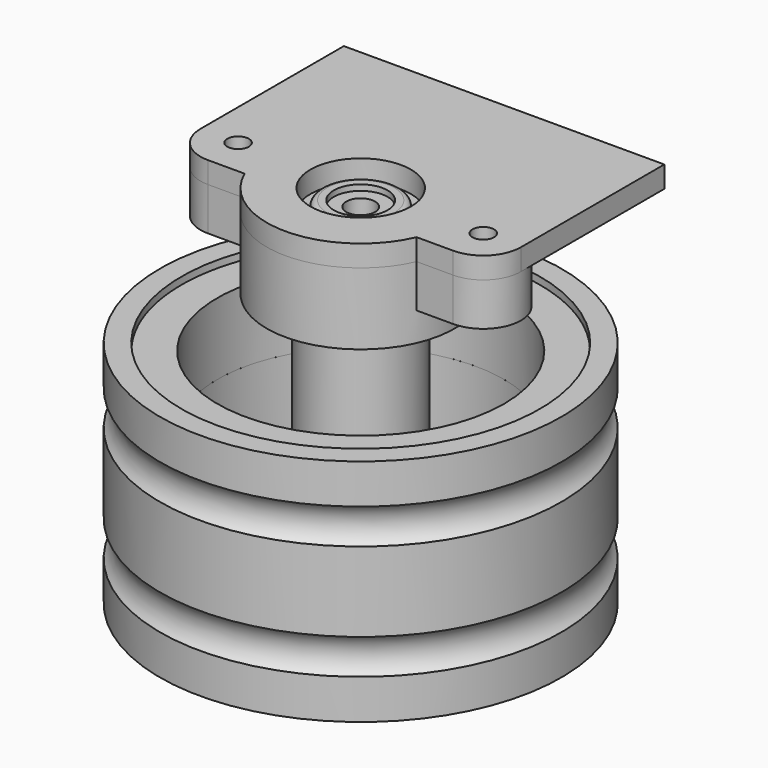
from build123d import *

# Parameters (mm, degrees)
F4_R           = 7.5
F4_R_2         = 3.75
F4_R_3         = 2.25
F5_DEPTH       = 10
F6_DEPTH       = 7.5
F9_W           = 2.45
F9_H           = 5
F11_R          = 0.2
F11_2_R        = 0.2
F12_R          = 0.6
F12_2_R        = 0.6
F13_R          = 0.8
F18_R          = 3.75
F18_R_2        = 2
F19_DEPTH      = 2
F20_DEPTH      = 6
F22_COUNT      = 2
F2_W           = 2
F2_H           = 5
F27_R          = 1.5
F28_REACH      = 54.2436406871
F31_END_RADIUS = 20
F30_R          = 3.5
F30_R_2        = 1.5
F31_REACH      = 16.9004949366
F27_R_2        = 2
F35_R          = 2
F36_DEPTH      = 47.1000001314
F38_DEPTH      = 4
F41_DEPTH      = 1
F42_R          = 2
F42_R_2        = 1.5
F43_DEPTH      = 3
F46_R          = 1


# Not quite as in the source:
# - a feature names something its author has since deleted; it is built from what else it names


with BuildPart() as f5:
    # F4 (on Top) → F5 (new body)
    with BuildSketch(Plane.XY):
        Circle(F4_R)
        Circle(F4_R_2, mode=Mode.SUBTRACT)
        Circle(F4_R_2)
        Circle(F4_R_3, mode=Mode.SUBTRACT)
    extrude(amount=F5_DEPTH)

    # F4 (on Top) → F6 (cut)
    with BuildSketch(Plane.XY):
        Circle(F4_R_2)
        Circle(F4_R_3, mode=Mode.SUBTRACT)
    extrude(amount=F6_DEPTH, mode=Mode.SUBTRACT)

    # F7 (on Front) → F8 (revolve)
    with BuildSketch(Plane.XZ):
        Polygon((-4.875, 12), (-6.0297005384, 10), (-3.7202994616, 10), align=None)
    revolve(axis=Axis((0, 0, 0), (0, 0, -1)))

    # F11
    f11_edges = [f5.edges().sort_by_distance(p)[0] for p in [
        (4.875, 0, 12),
    ]]
    fillet(f11_edges, radius=F11_R)

    # F12
    f12_edges = [f5.edges().sort_by_distance(p)[0] for p in [
        (-2.25, 0, 7.5),
        (-3.75, 0, 7.5),
    ]]
    fillet(f12_edges, radius=F12_R)



with BuildPart() as f10:
    # F9 (on Front) → F10 (revolve)
    with BuildSketch(Plane.XZ):
        Polygon((1.5, 20), (1.5, 10), (3.6048294078, 10), (4.875, 12.2), (6.1451705922, 10), (7.5, 10), (7.5, 35.7358983849), (5.5, 39.2), (5.5, 40), (3.95, 40), (1.5, 40), (1.5, 37), (0, 37), (0, 20), align=None)
        with Locations((2.725, 42.5)):
            Rectangle(F9_W, F9_H)
    revolve(axis=Axis((0, 0, 27.5), (0, 0, 1)))

    # F11#2
    f11_2_edges = [f10.edges().sort_by_distance(p)[0] for p in [
        (-4.875, 0, 12.2),
    ]]
    fillet(f11_2_edges, radius=F11_2_R)

    # F12#2
    f12_2_edges = [f10.edges().sort_by_distance(p)[0] for p in [
        (-1.5, 0, 20),
    ]]
    fillet(f12_2_edges, radius=F12_2_R)


with BuildPart() as f10b:
    # F9 (on Front) → F10, piece 2 (revolve)
    with BuildSketch(Plane.XZ):
        Polygon((2, 45.2), (3.95, 45.2), (3.95, 47), (5.5, 47), (5.5, 48.5), (3.75, 48.5), (3.75, 47.7), (2, 47.7), align=None)
    revolve(axis=Axis((0, 0, 27.5), (0, 0, 1)))

    # F13
    f13_edges = [f10b.edges().sort_by_distance(p)[0] for p in [
        (-5.5, 0, 48.5),
    ]]
    fillet(f13_edges, radius=F13_R)


with BuildPart() as f15:
    # F14 (on Front) → F15 (revolve)
    with BuildSketch(Plane.XZ):
        Polygon((-5.5, 40), (-5.5, 47), (-11, 47), (-11, 43.5), (-11, 40), align=None)
        Polygon((-4, 47), (-5.5, 47), (-5.5, 40), (-4, 40), (-4, 43.5), align=None)
    revolve(axis=Axis((0, 0, 43.5), (0, 0, 1)))


with BuildPart() as f17:
    # F16 (on Front) → F17 (revolve)
    with BuildSketch(Plane.XZ):
        Polygon((-7, 38.5), (-7, 40), (-11.1, 40), (-11.1, 47), (-13.1, 47), (-13.1, 44), (-13.1, 37), (-7.8660254038, 37), align=None)
    revolve(axis=Axis((0, 0, 42.5), (0, 0, -1)))

    # F18 (on face) → F19 (join)
    with BuildSketch(Plane.XY.offset(47)):
        with BuildLine():
            ThreePointArc((-12.7619152047, 2.956944421), (-14.6465797557, 4.6414684212), (-17.1, 5.25))
            ThreePointArc((-17.1, 5.25), (-22.35, 0), (-17.1, -5.25))
            ThreePointArc((-17.1, -5.25), (-14.6465797557, -4.6414684212), (-12.7619152047, -2.956944421))
            ThreePointArc((-12.7619152047, -2.956944421), (-13.1, 0), (-12.7619152047, 2.956944421))
        make_face()
        with Locations((-17.1, 0)):
            Circle(F18_R, mode=Mode.SUBTRACT)
        with Locations((-17.1, 0)):
            Circle(F18_R)
        with Locations((-17.1, 0)):
            Circle(F18_R_2, mode=Mode.SUBTRACT)
        with BuildLine():
            ThreePointArc((-12.7619152047, -2.956944421), (-14.6465797557, -4.6414684212), (-17.1, -5.25))
            Line((-17.1, -5.25), (-12.0019790035, -5.25))
            ThreePointArc((-12.0019790035, -5.25), (-12.4349161662, -4.1210265638), (-12.7619152047, -2.956944421))
        make_face()
        with BuildLine():
            Line((-12.0019790035, 5.25), (-17.1, 5.25))
            ThreePointArc((-17.1, 5.25), (-14.6465797557, 4.6414684212), (-12.7619152047, 2.956944421))
            ThreePointArc((-12.7619152047, 2.956944421), (-12.4349161662, 4.1210265638), (-12.0019790035, 5.25))
        make_face()
    extrude(amount=-F19_DEPTH)

    # F18 (on face) → F20 (join)
    with BuildSketch(Plane.XY.offset(47)):
        with BuildLine():
            ThreePointArc((-12.7619152047, 2.956944421), (-14.6465797557, 4.6414684212), (-17.1, 5.25))
            ThreePointArc((-17.1, 5.25), (-22.35, 0), (-17.1, -5.25))
            ThreePointArc((-17.1, -5.25), (-14.6465797557, -4.6414684212), (-12.7619152047, -2.956944421))
            ThreePointArc((-12.7619152047, -2.956944421), (-13.1, 0), (-12.7619152047, 2.956944421))
        make_face()
        with Locations((-17.1, 0)):
            Circle(F18_R, mode=Mode.SUBTRACT)
        with BuildLine():
            Line((-12.0019790035, 5.25), (-17.1, 5.25))
            ThreePointArc((-17.1, 5.25), (-14.6465797557, 4.6414684212), (-12.7619152047, 2.956944421))
            ThreePointArc((-12.7619152047, 2.956944421), (-12.4349161662, 4.1210265638), (-12.0019790035, 5.25))
        make_face()
        with BuildLine():
            ThreePointArc((-12.7619152047, -2.956944421), (-14.6465797557, -4.6414684212), (-17.1, -5.25))
            Line((-17.1, -5.25), (-12.0019790035, -5.25))
            ThreePointArc((-12.0019790035, -5.25), (-12.4349161662, -4.1210265638), (-12.7619152047, -2.956944421))
        make_face()
    extrude(amount=-F20_DEPTH)

    # F21: union 


with BuildPart() as f22_1:
    # F22: instance of F17
    add(f17.part.rotate(Axis((0, 0, 42.5), (0, 0, -1)), 1 * 360 / F22_COUNT))


with BuildPart() as f17_1:
    add(f17.part)

    # F23: union F22_1
    add(f22_1.part)

    # F46
    f46_edges = [f17_1.edges().sort_by_distance(p)[0] for p in [
        (11.1, 0, 47),
    ]]
    fillet(f46_edges, radius=F46_R)


with BuildPart() as f24:
    # F1 (on Front) + F2 (on Front) → F24 (revolve)
    with BuildSketch(Plane.XZ):
        Polygon((25, 0), (25, 5), (23, 5), (23, 15), (20, 15), (20, 0), align=None)
    with BuildSketch(Plane.XZ):
        with Locations((21, 17.5)):
            Rectangle(F2_W, F2_H)
    revolve(axis=Axis((0, 0, 0), (0, 0, -1)))

    # F25: union 

    f28_end = f10.part.faces().sort_by_distance((-7.5, 0, 22.8679491924))[0]
    # F27 (on offset) → F28 (cut, up to a face of F10 that its end follows)
    with BuildSketch(Plane.XZ.offset(25)):
        with Locations((0, 17.5)):
            Circle(F27_R)
    f28_long = extrude(amount=-F28_REACH, mode=Mode.PRIVATE)
    add(split(f28_long, bisect_by=f28_end, keep=Keep.ALL, mode=Mode.PRIVATE).solids().sort_by_distance((0, -25, 17.5))[0], mode=Mode.SUBTRACT)

    f31_end = (Plane(origin=(0, 0, 10), x_dir=(-1, 0, 0), z_dir=(0, 0, -1)) * Cylinder(F31_END_RADIUS, 205.2915145059, mode=Mode.PRIVATE)).faces().sort_by_distance((-20, 0, 10))[0]
    # F30 (on offset) → F31 (join, up to the whole of a round face its end follows)
    with BuildSketch(Plane.XZ.offset(18)):
        with Locations((0, 17.5)):
            Circle(F30_R)
        with Locations((0, 17.5)):
            Circle(F30_R_2, mode=Mode.SUBTRACT)
    f31_long = extrude(amount=F31_REACH, mode=Mode.PRIVATE)
    add(split(f31_long, bisect_by=f31_end, keep=Keep.BOTTOM, mode=Mode.PRIVATE))

    # F32 (on Right) → F33 (revolve, cut)
    with BuildSketch(Plane.YZ):
        Polygon((-19, 21), (-20, 21), (-20, 20), align=None)
    revolve(axis=Axis((0, 0, 15), (0, 0, -1)), mode=Mode.SUBTRACT)


with BuildPart() as f34:
    # F3 (on Front) → F34 (revolve)
    with BuildSketch(Plane.XZ):
        Polygon((25, 30), (20, 30), (20, 20), (22.2, 20), (22.2, 15), (23, 15), (23, 25), (25, 25), align=None)
    revolve(axis=Axis((0, 0, 0), (0, 0, -1)))

    # F27 (on offset) + F35 (on offset) → F36 (cut, up to face)
    with BuildSketch(Plane.XZ.offset(25)):
        with Locations((0, 17.5)):
            Circle(F27_R_2)
        with Locations((0, 17.5)):
            Circle(F27_R, mode=Mode.SUBTRACT)
    with BuildSketch(Plane.XZ.offset(25)):
        with Locations((0, 17.5)):
            Circle(F35_R)
    extrude(amount=-F36_DEPTH, mode=Mode.SUBTRACT)


with BuildPart() as f5_1:
    add(f5.part)

    add(f24.part)  # F38 merges F24
    # F37 (on face) → F38 (join)
    with BuildSketch(Plane.XY):
        with BuildLine():
            ThreePointArc((-3.0067767078, -19.7726906067), (0, -20), (3.0067767078, -19.7726906067))
            Line((3.0067767078, -19.7726906067), (5, -5.5901699437))
            ThreePointArc((5, -5.5901699437), (0, -7.5), (-5, -5.5901699437))
            Line((-5, -5.5901699437), (-3.0067767078, -19.7726906067))
        make_face()
        with BuildLine():
            Line((7.3412291828, -1.535042047), (18.6270407205, 7.2824002909))
            ThreePointArc((18.6270407205, 7.2824002909), (17.3205080757, 10), (15.6202640127, 12.4902903159))
            Line((15.6202640127, 12.4902903159), (2.3412291828, 7.1252119908))
            ThreePointArc((2.3412291828, 7.1252119908), (6.0749164139, 4.3983395236), (7.5, 0))
            ThreePointArc((7.5, 0), (7.4602017021, -0.771615555), (7.3412291828, -1.535042047))
        make_face()
        with BuildLine():
            Line((-18.6270407205, 7.2824002909), (-7.3412291828, -1.535042047))
            ThreePointArc((-7.3412291828, -1.535042047), (-6.4951905284, 3.75), (-2.3412291828, 7.1252119908))
            Line((-2.3412291828, 7.1252119908), (-15.6202640127, 12.4902903159))
            ThreePointArc((-15.6202640127, 12.4902903159), (-17.3205080757, 10), (-18.6270407205, 7.2824002909))
        make_face()
    extrude(amount=F38_DEPTH)

    # F39: union 

    # F40 (on face) → F41 (cut)
    with BuildSketch(Plane(origin=(0, 0, 0), x_dir=(1, 0, 0), z_dir=(0, 0, -1))):
        with BuildLine():
            ThreePointArc((-18.6270407205, -7.2824002909), (-17.3205080757, -10), (-15.6202640127, -12.4902903159))
            Line((-15.6202640127, -12.4902903159), (-14.6502345253, -12.0983729631))
            ThreePointArc((-14.6502345253, -12.0983729631), (-16.4544826719, -9.5), (-17.8026155932, -6.6382887887))
            Line((-17.8026155932, -6.6382887887), (-18.6270407205, -7.2824002909))
        make_face()
        with BuildLine():
            Line((14.6502345253, -12.0983729631), (15.6202640127, -12.4902903159))
            ThreePointArc((15.6202640127, -12.4902903159), (17.3205080757, -10), (18.6270407205, -7.2824002909))
            Line((18.6270407205, -7.2824002909), (17.8026155932, -6.6382887887))
            ThreePointArc((17.8026155932, -6.6382887887), (16.4544826719, -9.5), (14.6502345253, -12.0983729631))
        make_face()
        with BuildLine():
            ThreePointArc((-8.4751793611, 0.6491030715), (-7.3612159322, -4.25), (-3.6754499309, -7.6642721641))
            Line((-3.6754499309, -7.6642721641), (-2.3412291828, -7.1252119908))
            ThreePointArc((-2.3412291828, -7.1252119908), (-6.4951905284, -3.75), (-7.3412291828, 1.535042047))
            Line((-7.3412291828, 1.535042047), (-8.4751793611, 0.6491030715))
        make_face()
        with BuildLine():
            Line((2.3412291828, -7.1252119908), (3.6754499309, -7.6642721641))
            ThreePointArc((3.6754499309, -7.6642721641), (7.1934457811, -4.5281715729), (8.5, 0))
            ThreePointArc((8.5, 0), (8.4937925737, 0.3247887243), (8.4751793611, 0.6491030715))
            Line((8.4751793611, 0.6491030715), (7.3412291828, 1.535042047))
            ThreePointArc((7.3412291828, 1.535042047), (7.4602017021, 0.771615555), (7.5, 0))
            ThreePointArc((7.5, 0), (6.0749164139, -4.3983395236), (2.3412291828, -7.1252119908))
        make_face()
        with BuildLine():
            ThreePointArc((3.0067767078, 19.7726906067), (0, 20), (-3.0067767078, 19.7726906067))
            Line((-3.0067767078, 19.7726906067), (-3.1523810679, 18.7366617518))
            ThreePointArc((-3.1523810679, 18.7366617518), (0, 19), (3.1523810679, 18.7366617518))
            Line((3.1523810679, 18.7366617518), (3.0067767078, 19.7726906067))
        make_face()
        with BuildLine():
            ThreePointArc((4.7997294302, 7.0151690926), (0, 8.5), (-4.7997294302, 7.0151690926))
            Line((-4.7997294302, 7.0151690926), (-5, 5.5901699437))
            ThreePointArc((-5, 5.5901699437), (0, 7.5), (5, 5.5901699437))
            Line((5, 5.5901699437), (4.7997294302, 7.0151690926))
        make_face()
    extrude(amount=-F41_DEPTH, mode=Mode.SUBTRACT)


with BuildPart() as f43:
    # F42 (on face) → F43 (new body)
    with BuildSketch(Plane.XY.offset(47)):
        with BuildLine():
            Line((-17.1, -5.25), (-12.0019790035, -5.25))
            Line((-12.0019790035, -5.25), (-9.7799539876, -5.25))
            ThreePointArc((-9.7799539876, -5.25), (-2.7067056302, 10.7649312414), (11.1, 0))
            ThreePointArc((11.1, 0), (10.7649312414, -2.7067056302), (9.7799539876, -5.25))
            Line((9.7799539876, -5.25), (12.0019790035, -5.25))
            Line((12.0019790035, -5.25), (17.1, -5.25))
            ThreePointArc((17.1, -5.25), (20.8123106012, -3.7123106012), (22.35, 0))
            ThreePointArc((22.35, 0), (20.8123106012, 3.7123106012), (17.1, 5.25))
            Line((17.1, 5.25), (12.0019790035, 5.25))
            ThreePointArc((12.0019790035, 5.25), (0, 13.1), (-12.0019790035, 5.25))
            Line((-12.0019790035, 5.25), (-17.1, 5.25))
            ThreePointArc((-17.1, 5.25), (-20.8123106012, 3.7123106012), (-22.35, 0))
            ThreePointArc((-22.35, 0), (-20.8123106012, -3.7123106012), (-17.1, -5.25))
        make_face()
        with Locations((-17.1, 0)):
            Circle(F42_R, mode=Mode.SUBTRACT)
        with Locations((17.1, 0)):
            Circle(F42_R, mode=Mode.SUBTRACT)
        with BuildLine():
            Line((-22.35, 25), (-22.35, 0))
            ThreePointArc((-22.35, 0), (-20.8123106012, 3.7123106012), (-17.1, 5.25))
            Line((-17.1, 5.25), (-12.0019790035, 5.25))
            ThreePointArc((-12.0019790035, 5.25), (0, 13.1), (12.0019790035, 5.25))
            Line((12.0019790035, 5.25), (17.1, 5.25))
            ThreePointArc((17.1, 5.25), (20.8123106012, 3.7123106012), (22.35, 0))
            Line((22.35, 0), (22.35, 25))
            Line((22.35, 25), (-22.35, 25))
        make_face()
        with BuildLine():
            ThreePointArc((11.1, 0), (-2.7067056302, 10.7649312414), (-9.7799539876, -5.25))
            Line((-9.7799539876, -5.25), (-4.6300647944, -5.25))
            ThreePointArc((-4.6300647944, -5.25), (-2.8800647944, 6.3800647944), (7, 0))
            ThreePointArc((7, 0), (6.3800647944, -2.8800647944), (4.6300647944, -5.25))
            Line((4.6300647944, -5.25), (9.7799539876, -5.25))
            ThreePointArc((9.7799539876, -5.25), (10.7649312414, -2.7067056302), (11.1, 0))
        make_face()
        with BuildLine():
            Line((-4.6300647944, -5.25), (-9.7799539876, -5.25))
            ThreePointArc((-9.7799539876, -5.25), (0, -11.1), (9.7799539876, -5.25))
            Line((9.7799539876, -5.25), (4.6300647944, -5.25))
            ThreePointArc((4.6300647944, -5.25), (0, -7), (-4.6300647944, -5.25))
        make_face()
        with BuildLine():
            Line((-9.7799539876, -5.25), (-12.0019790035, -5.25))
            ThreePointArc((-12.0019790035, -5.25), (0, -13.1), (12.0019790035, -5.25))
            Line((12.0019790035, -5.25), (9.7799539876, -5.25))
            ThreePointArc((9.7799539876, -5.25), (0, -11.1), (-9.7799539876, -5.25))
        make_face()
        with Locations((-17.1, 0)):
            Circle(F42_R)
        with Locations((-17.1, 0)):
            Circle(F42_R_2, mode=Mode.SUBTRACT)
        with Locations((17.1, 0)):
            Circle(F42_R)
        with Locations((17.1, 0)):
            Circle(F42_R_2, mode=Mode.SUBTRACT)
    extrude(amount=F43_DEPTH)


with BuildPart() as f45:
    # F44 (on Right) → F45 (revolve)
    with BuildSketch(Plane.YZ):
        with BuildLine():
            Line((25, 25), (23, 25))
            Line((23, 25), (23, 22.5))
            ThreePointArc((23, 22.5), (26.3856217223, 15), (23, 7.5))
            Line((23, 7.5), (23, 5))
            Line((23, 5), (25, 5))
            Line((25, 5), (25, 0))
            Line((25, 0), (25, -1))
            Line((25, -1), (28, -1))
            Line((28, -1), (28, 4.5505102572))
            ThreePointArc((28, 4.5505102572), (27, 7), (28, 9.4494897428))
            Line((28, 9.4494897428), (28, 20.5505102572))
            ThreePointArc((28, 20.5505102572), (27, 23), (28, 25.4494897428))
            Line((28, 25.4494897428), (28, 31))
            Line((28, 31), (25, 31))
            Line((25, 31), (25, 30))
            Line((25, 30), (25, 25))
        make_face()
    revolve(axis=Axis((0, 0, 15), (0, 0, -1)))


solid = Compound([f10.part, f10b.part, f15.part, f17_1.part, f34.part, f5_1.part, f43.part, f45.part])
